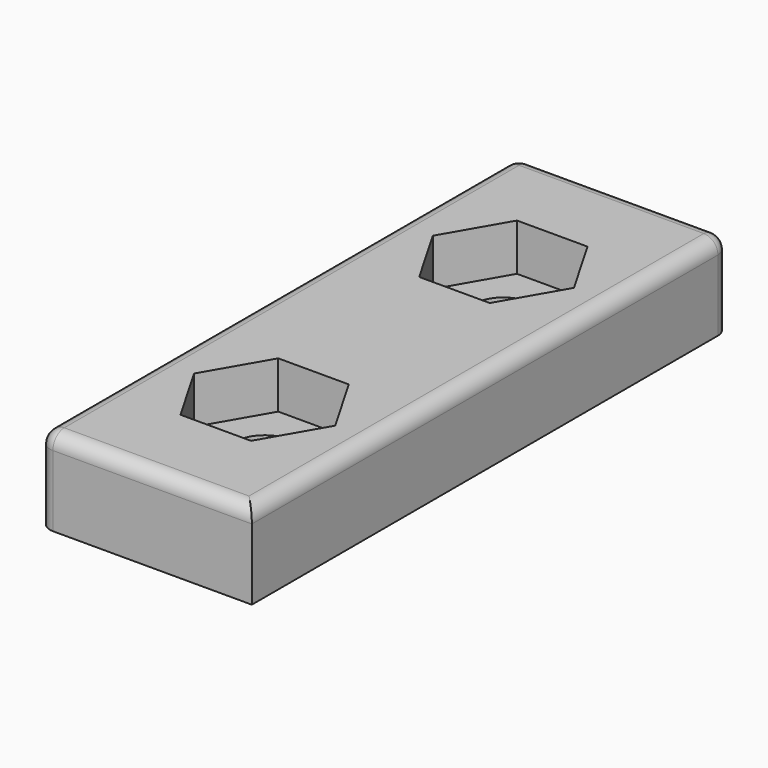
from build123d import *

# Parameters (mm, degrees)
F0_W     = 15
F0_H     = 42
F0_R     = 2.1
F1_DEPTH = 6
F2_DEPTH = 6.001
F3_R     = 2.1
F4_DEPTH = 3.3
F5_R     = 1


# Not quite as in the source:
# - a feature names something its author has since deleted; it is built from what else it names


with BuildPart() as f1:
    # F0 (on Top) → F1 (new body)
    with BuildSketch(Plane.XY):
        Rectangle(F0_W, F0_H)
        with Locations((0, -10.5)):
            Circle(F0_R, mode=Mode.SUBTRACT)
        with Locations((0, 10.5)):
            Circle(F0_R, mode=Mode.SUBTRACT)
        with Locations((0, -10.5)):
            Circle(F0_R)
        with Locations((0, 10.5)):
            Circle(F0_R)
    extrude(amount=F1_DEPTH)

    # F0 (on Top) → F2 (cut, through all)
    with BuildSketch(Plane.XY):
        with Locations((0, 10.5)):
            Circle(F0_R)
        with Locations((0, -10.5)):
            Circle(F0_R)
    extrude(amount=F2_DEPTH, mode=Mode.SUBTRACT)

    # F3 (on face) → F4 (cut)
    with BuildSketch(Plane.XY.offset(6)):
        Polygon((4.965212315, -10.5), (2.4826061575, -6.2), (-2.4826061575, -6.2), (-4.965212315, -10.5), (-2.4826061575, -14.8), (2.4826061575, -14.8), align=None)
        with Locations((0, -10.5)):
            Circle(F3_R, mode=Mode.SUBTRACT)
        Polygon((4.965212315, 10.5), (2.4826061575, 14.8), (-2.4826061575, 14.8), (-4.965212315, 10.5), (-2.4826061575, 6.2), (2.4826061575, 6.2), align=None)
        with Locations((0, 10.5)):
            Circle(F3_R, mode=Mode.SUBTRACT)
    extrude(amount=-F4_DEPTH, mode=Mode.SUBTRACT)

    # F5
    f5_edges = [f1.edges().sort_by_distance(p)[0] for p in [
        (-7.5, 21, 3),
        (-7.5, -21, 3),
        (0, -21, 6),
        (-7.5, 0, 6),
        (0, 21, 6),
        (7.5, 0, 6),
        (7.5, 21, 3),
    ]]
    fillet(f5_edges, radius=F5_R)


solid = f1.part
